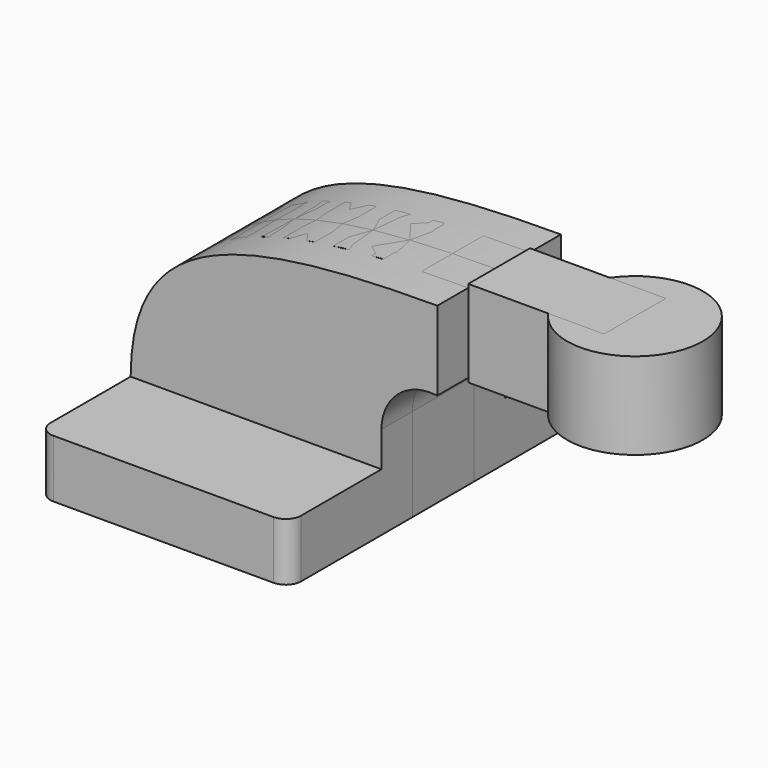
from build123d import *

# Parameters (mm, degrees)
F0_W     = 82.55
F0_H     = 19.05
F1_DEPTH = 63.5
F2_DEPTH = 25.4
F4_R     = 5.08
F0_W_2   = 22.3502442241
F0_H_2   = 26.0258951836
F0_H_3   = 1.1622799838
F0_H_4   = 1.3868248326
F5_DEPTH = 12.7


# Not quite as in the source:
# - a feature names something its author has since deleted; it is built from what else it names


with BuildPart() as f1:
    # F0 (on Front) → F1 (new body, symmetric)
    with BuildSketch(Plane.XZ):
        Rectangle(F0_W, F0_H)
    extrude(amount=F1_DEPTH, both=True)

    # F0 (on Front) → F2 (join, symmetric)
    with BuildSketch(Plane.XZ):
        with BuildLine():
            add(Edge.make_bspline(
                [(-41.275, 9.525), (-41.0884097219, 53.2467439771), (-7.776630111, 62.8007799387), (59.6824064851, 62.9030779754)],
                knots=[0, 0, 0, 0, 114.1998998798, 114.1998998798, 114.1998998798, 114.1998998798], degree=3))
            Line((-41.275, 9.525), (41.275, 9.525))
            Line((41.275, 9.525), (41.275, 21.0693579674))
            ThreePointArc((41.275, 21.0693579674), (46.5551227902, 32.9028879626), (58.8886992965, 36.8771827918))
            Line((58.8886992965, 36.8771827918), (59.6824064851, 36.8771827918))
            Line((59.6824064851, 36.8771827918), (59.6824064851, 62.9030779754))
        make_face()
    extrude(amount=F2_DEPTH, both=True)

    # F4
    f4_edges = [f1.edges().sort_by_distance(p)[0] for p in [
        (41.275, -63.5, 0),
        (-41.275, -63.5, 0),
        (41.275, 63.5, 0),
        (-41.275, 63.5, 0),
    ]]
    fillet(f4_edges, radius=F4_R)


with BuildPart() as f3:
    # F0 (on Front) → F3 (revolve)
    with BuildSketch(Plane.XZ):
        Polygon((82.0326507092, 64.0653579593), (82.0326507092, 62.9030779754), (82.0326507092, 36.8771827918), (82.0326507092, 35.4903579593), (104.3828949332, 35.4903579593), (104.3828949332, 64.0653579593), align=None)
    revolve(axis=Axis((104.3828949332, 0, 49.7778579593), (0, 0, 1)))


with BuildPart() as f5:
    # F0 (on Front) → F5 (new body, symmetric)
    with BuildSketch(Plane.XZ):
        Rectangle(F0_W, F0_H)
        with BuildLine():
            add(Edge.make_bspline(
                [(-41.275, 9.525), (-41.0884097219, 53.2467439771), (-7.776630111, 62.8007799387), (59.6824064851, 62.9030779754)],
                knots=[0, 0, 0, 0, 114.1998998798, 114.1998998798, 114.1998998798, 114.1998998798], degree=3))
            Line((-41.275, 9.525), (41.275, 9.525))
            Line((41.275, 9.525), (41.275, 21.0693579674))
            ThreePointArc((41.275, 21.0693579674), (46.5551227902, 32.9028879626), (58.8886992965, 36.8771827918))
            Line((58.8886992965, 36.8771827918), (59.6824064851, 36.8771827918))
            Line((59.6824064851, 36.8771827918), (59.6824064851, 62.9030779754))
        make_face()
        with Locations((70.8575285971, 49.8901303836)):
            Rectangle(F0_W_2, F0_H_2)
        with Locations((70.8575285971, 63.4842179674)):
            Rectangle(F0_W_2, F0_H_3)
        with Locations((70.8575285971, 36.1837703755)):
            Rectangle(F0_W_2, F0_H_4)
        Polygon((82.0326507092, 64.0653579593), (82.0326507092, 62.9030779754), (82.0326507092, 36.8771827918), (82.0326507092, 35.4903579593), (104.3828949332, 35.4903579593), (104.3828949332, 64.0653579593), align=None)
    extrude(amount=F5_DEPTH, both=True)


solid = Compound([f1.part, f3.part, f5.part])
